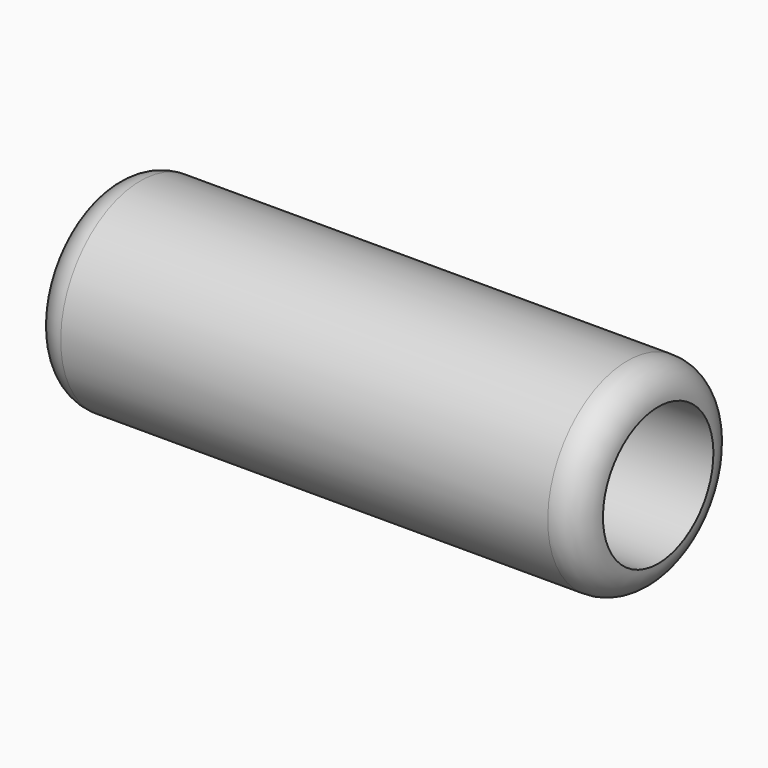
from build123d import *

# Parameters (mm, degrees)
F2_R = 6.34999


# Not quite as in the source:
# - a fillet or chamfer is up to 0.001 mm smaller than in the source, because OpenCascade refuses the exact size


with BuildPart() as f1:
    # F0 (on Front) → F1 (revolve)
    with BuildSketch(Plane.XZ):
        Polygon((-48.2103834725, -19.5578883292), (-48.2103834725, -35.4328883292), (65.3022165275, -35.4328883292), (65.3022165275, -29.0828883292), (-44.2479834725, -29.0828883292), (-44.2479834725, -19.5578883292), align=None)
    revolve(axis=Axis((10.06000489, 0, -14.7953883292), (1, 0, 0)))

    # F2 (radius 6.35 in the source; OpenCascade refuses exactly that, so slightly less here)
    f2_edges = [f1.edges().sort_by_distance(p)[0] for p in [
        (-48.210383, 0, 5.842112),
        (65.302217, 0, 5.842112),
    ]]
    fillet(f2_edges, radius=F2_R)


solid = f1.part
